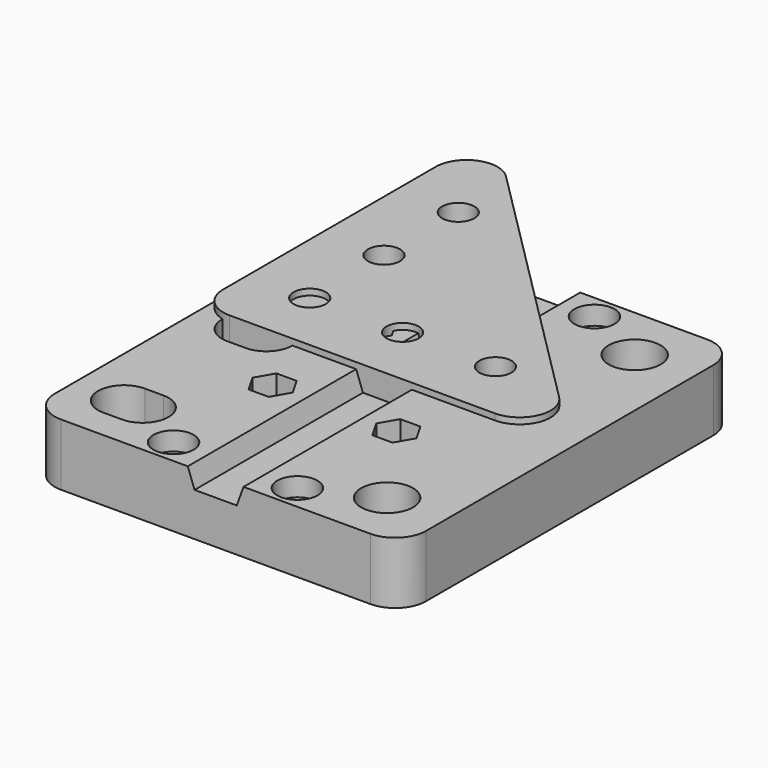
from build123d import *

# Parameters (mm, degrees)
F0_R           = 2.6
F1_DEPTH       = 6
F2_R           = 5
F3_W           = 60
F3_H           = 68
F3_R           = 4.2
F4_DEPTH       = 5
F5_R           = 5
F7_D           = 3.3
F7_CBORE_D     = 6.5
F7_CBORE_DEPTH = 3
F9_DEPTH       = 4
F10_D          = 3.3
F12_DEPTH      = 3
F12_TAPER      = 20
F13_DEPTH      = 68.001


with BuildPart() as f1:
    # F0 (on Top) → F1 (new body)
    with BuildSketch(Plane.XY):
        Polygon((-30, 60), (-30, 0), (30, 0), align=None)
        with Locations((-20, 10)):
            Circle(F0_R, mode=Mode.SUBTRACT)
        with Locations((-5, 10)):
            Circle(F0_R, mode=Mode.SUBTRACT)
        with Locations((-20, 25)):
            Circle(F0_R, mode=Mode.SUBTRACT)
        with Locations((10, 10)):
            Circle(F0_R, mode=Mode.SUBTRACT)
        with Locations((-20, 40)):
            Circle(F0_R, mode=Mode.SUBTRACT)
    extrude(amount=F1_DEPTH)

    # F2
    f2_edges = [f1.edges().sort_by_distance(p)[0] for p in [
        (-30, 0, 3),
        (30, 0, 3),
        (-30, 60, 3),
    ]]
    fillet(f2_edges, radius=F2_R)


with BuildPart() as f4:
    # F3 (on Top) → F4 (new body, symmetric)
    with BuildSketch(Plane.XY):
        Rectangle(F3_W, F3_H)
        with BuildLine():
            ThreePointArc((-19, -20.8), (-14.8, -25), (-19, -29.2))
            Line((-19, -29.2), (-22, -29.2))
            ThreePointArc((-22, -29.2), (-26.2, -25), (-22, -20.8))
            Line((-22, -20.8), (-19, -20.8))
        make_face(mode=Mode.SUBTRACT)
        with Locations((20.5, -25)):
            Circle(F3_R, mode=Mode.SUBTRACT)
        with BuildLine():
            ThreePointArc((-19, 4.2), (-14.8, 0), (-19, -4.2))
            Line((-19, -4.2), (-22, -4.2))
            ThreePointArc((-22, -4.2), (-26.2, 0), (-22, 4.2))
            Line((-22, 4.2), (-19, 4.2))
        make_face(mode=Mode.SUBTRACT)
        with BuildLine():
            ThreePointArc((-19, 29.2), (-14.8, 25), (-19, 20.8))
            Line((-19, 20.8), (-22, 20.8))
            ThreePointArc((-22, 20.8), (-26.2, 25), (-22, 29.2))
            Line((-22, 29.2), (-19, 29.2))
        make_face(mode=Mode.SUBTRACT)
        with Locations((20.5, 25)):
            Circle(F3_R, mode=Mode.SUBTRACT)
    extrude(amount=F4_DEPTH, both=True)

    # F5
    f5_edges = [f4.edges().sort_by_distance(p)[0] for p in [
        (-30, 34, 0),
        (-30, -34, 0),
        (30, -34, 0),
        (30, 34, 0),
    ]]
    fillet(f5_edges, radius=F5_R)

    # F7 (through all)
    with Locations(Plane.XY.offset(5)):
        with Locations((-10, 30), (10, 30), (-10, -30), (10, -30)):
            CounterBoreHole(F7_D / 2, F7_CBORE_D / 2, F7_CBORE_DEPTH)

    # F8 (on face) → F9 (cut)
    with BuildSketch(Plane.XY.offset(5)):
        Polygon((-11.625, 12.8145825623), (-13.25, 10), (-11.625, 7.1854174377), (-8.375, 7.1854174377), (-6.75, 10), (-8.375, 12.8145825623), align=None)
        Polygon((8.375, 12.8145825623), (6.75, 10), (8.375, 7.1854174377), (11.625, 7.1854174377), (13.25, 10), (11.625, 12.8145825623), align=None)
        Polygon((-8.375, -12.8145825623), (-6.75, -10), (-8.375, -7.1854174377), (-11.625, -7.1854174377), (-13.25, -10), (-11.625, -12.8145825623), align=None)
        Polygon((8.375, -7.1854174377), (6.75, -10), (8.375, -12.8145825623), (11.625, -12.8145825623), (13.25, -10), (11.625, -7.1854174377), align=None)
    extrude(amount=-F9_DEPTH, mode=Mode.SUBTRACT)

    # F10 (through all)
    with Locations(Plane.XY.offset(5)):
        with Locations((-10, 10), (10, 10), (-10, -10), (10, -10)):
            Hole(F10_D / 2)

    # F11 (on face) → F12 (cut)
    with BuildSketch(Plane(origin=(0, 34, 0), x_dir=(-1, 0, 0), z_dir=(0, 1, 0))):
        Polygon((4.5, 5), (-4.5, 5), (-3.4080892972, 2), (3.4080892972, 2), align=None)
    extrude(amount=-F12_DEPTH, taper=F12_TAPER, mode=Mode.SUBTRACT)

    # F11 (on face) → F13 (cut, through all)
    with BuildSketch(Plane(origin=(0, 34, 0), x_dir=(-1, 0, 0), z_dir=(0, 1, 0))):
        Polygon((4.5, 5), (-4.5, 5), (-3.4080892972, 2), (3.4080892972, 2), align=None)
    extrude(amount=-F13_DEPTH, mode=Mode.SUBTRACT)


solid = Compound([f1.part, f4.part])
